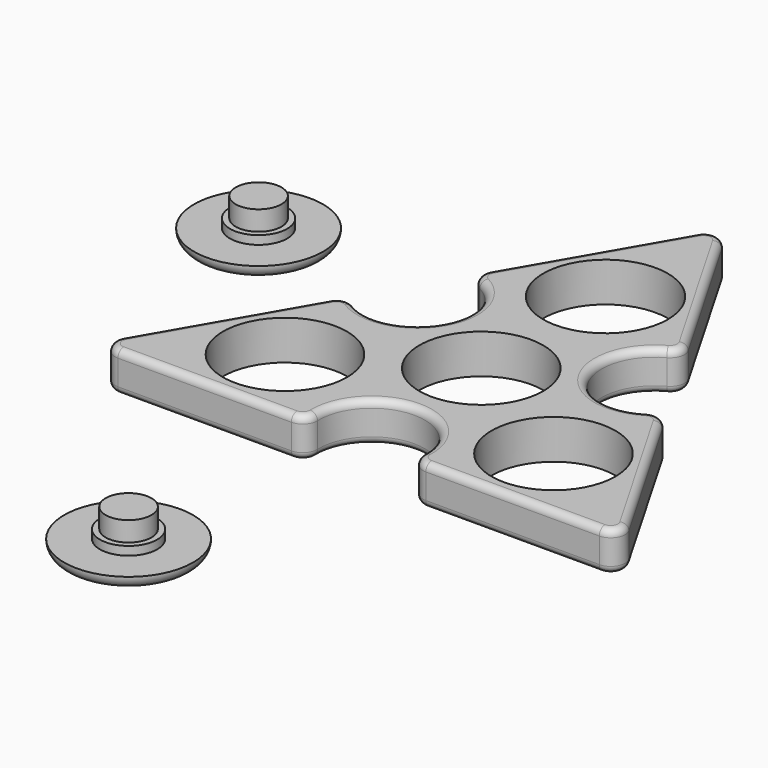
from build123d import *

# Parameters (mm, degrees)
F0_R         = 10.9982
F0_R_2       = 11.049
F1_DEPTH     = 7.0000114
F2_R         = 2.54
F3_R         = 11.43
F4_DEPTH     = 2.286
F5_R         = 2.28599
F7_TEXT_SIZE = 18.0475862133
F8_DEPTH     = 1.27
F9_TEXT_SIZE = 18.8806337371
F10_DEPTH    = 1.27
F11_R        = 5.08
F12_DEPTH    = 1.524
F13_R        = 5.08
F14_DEPTH    = 1.524
F15_R        = 4.064
F16_DEPTH    = 3.499993
F17_R        = 4.064
F18_DEPTH    = 3.499993
F19_R        = 1.27


# Not quite as in the source:
# - a fillet or chamfer is up to 0.001 mm smaller than in the source, because OpenCascade refuses the exact size
# - Text() gives the source's letters only with a copy of the font that has no kerning and outlines rounded to 1/6400 em; it was checked with that copy


with BuildPart() as f1:
    # F0 (on Top) → F1 (new body)
    with BuildSketch(Plane.XY):
        with BuildLine():
            ThreePointArc((28.0221413684, 21.0966697702), (12.9013627731, 22.68860527), (19.0830954868, 36.5795514084))
            Line((19.0830954868, 36.5795514084), (0, 69.6324423572))
            Line((0, 69.6324423572), (-19.0830954868, 36.5795514084))
            ThreePointArc((-19.0830954868, 36.5795514084), (-12.9013627731, 22.68860527), (-28.0221413684, 21.0966697702))
            Line((-28.0221413684, 21.0966697702), (-47.1052368552, -11.9562211786))
            Line((-47.1052368552, -11.9562211786), (-8.9390458817, -11.9562211786))
            ThreePointArc((-8.9390458817, -11.9562211786), (0, 0.3427894601), (8.9390458817, -11.9562211786))
            Line((8.9390458817, -11.9562211786), (47.1052368552, -11.9562211786))
            Line((47.1052368552, -11.9562211786), (28.0221413684, 21.0966697702))
        make_face()
        with Locations((-23.8228000124, 1.4859)):
            Circle(F0_R, mode=Mode.SUBTRACT)
        with Locations((23.8228000124, 1.4859)):
            Circle(F0_R, mode=Mode.SUBTRACT)
        with Locations((0, 15.24)):
            Circle(F0_R, mode=Mode.SUBTRACT)
        with Locations((0, 42.799)):
            Circle(F0_R_2, mode=Mode.SUBTRACT)
    extrude(amount=F1_DEPTH)

    # F2
    f2_edges = [f1.edges().sort_by_distance(p)[0] for p in [
        (47.105237, -11.956221, 3.500006),
        (8.939046, -11.956221, 3.500006),
        (-8.939046, -11.956221, 3.500006),
        (-47.105237, -11.956221, 3.500006),
        (-28.022141, 21.09667, 3.500006),
        (-19.083095, 36.579551, 3.500006),
        (0, 69.632442, 3.500006),
        (28.022141, 21.09667, 3.500006),
        (19.083095, 36.579551, 3.500006),
    ]]
    fillet(f2_edges, radius=F2_R)

    # F19
    f19_edges = [f1.edges().sort_by_distance(p)[0] for p in [
        (0, 0.342789, 7.000011),
        (0, 0.342789, 0),
    ]]
    fillet(f19_edges, radius=F19_R)


with BuildPart() as f4:
    # F3 (on Top) → F4 (new body)
    with BuildSketch(Plane.XY):
        with Locations((-56.0353733599, 35.8910113573)):
            Circle(F3_R)
    extrude(amount=F4_DEPTH)

    # F5 (radius 2.286 in the source; OpenCascade refuses exactly that, so slightly less here)
    f5_edges = [f4.edges().sort_by_distance(p)[0] for p in [
        (-67.465373, 35.891011, 0),
    ]]
    fillet(f5_edges, radius=F5_R)


with BuildPart() as f6_1:
    # F6: copy of F4
    add(f4.part.moved(Location((44.196, -84.074, 0))))

    # F9 (on face) → F10 (cut)
    with BuildSketch(Plane(origin=(0, 0, 0), x_dir=(1, 0, 0), z_dir=(0, 0, -1))):
        with Locations((-18.0401048027, 41.3093241244)):
            Text('P', F9_TEXT_SIZE, font='Open Sans', font_style=FontStyle.BOLD, text_align=(TextAlign.LEFT, TextAlign.BOTTOM))
    extrude(amount=-F10_DEPTH, mode=Mode.SUBTRACT)

    # F11 (on face) → F12 (join)
    with BuildSketch(Plane.XY.offset(2.286)):
        with Locations((-11.8393733599, -48.1829886427)):
            Circle(F11_R)
    extrude(amount=F12_DEPTH)

    # F15 (on face) → F16 (join)
    with BuildSketch(Plane.XY.offset(3.81)):
        with Locations((-11.8393733599, -48.1829886427)):
            Circle(F15_R)
    extrude(amount=F16_DEPTH)


with BuildPart() as f4_1:
    add(f4.part)

    # F7 (on face) → F8 (cut)
    with BuildSketch(Plane(origin=(0, 0, 0), x_dir=(1, 0, 0), z_dir=(0, 0, -1))):
        with Locations((-62.9251138239, -42.8732677474)):
            Text('G', F7_TEXT_SIZE, font='Open Sans', font_style=FontStyle.BOLD, text_align=(TextAlign.LEFT, TextAlign.BOTTOM))
    extrude(amount=-F8_DEPTH, mode=Mode.SUBTRACT)

    # F13 (on face) → F14 (join)
    with BuildSketch(Plane.XY.offset(2.286)):
        with Locations((-56.0353733599, 35.8910113573)):
            Circle(F13_R)
    extrude(amount=F14_DEPTH)

    # F17 (on face) → F18 (join)
    with BuildSketch(Plane.XY.offset(3.81)):
        with Locations((-56.0353733599, 35.8910113573)):
            Circle(F17_R)
    extrude(amount=F18_DEPTH)


solid = Compound([f1.part, f6_1.part, f4_1.part])
